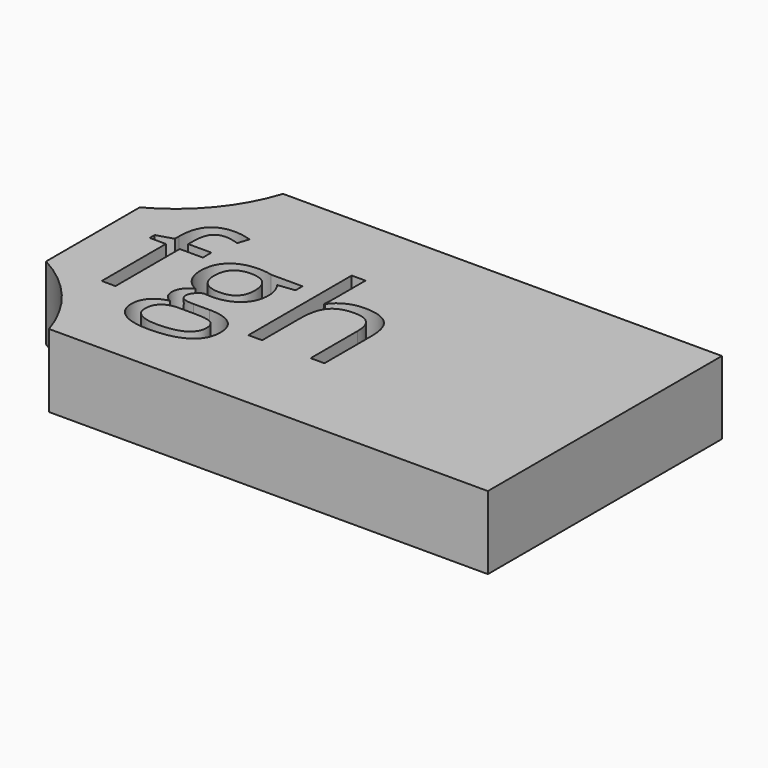
from build123d import *

# Parameters (mm, degrees)
F0_W         = 150
F0_H         = 100
F1_DEPTH     = 2
F2_DEPTH     = 25
F3_TEXT_SIZE = 58.1079033307
F4_DEPTH     = 25


# Not quite as in the source:
# - Text() gives the source's letters only with a copy of the font that has no kerning and outlines rounded to 1/6400 em; it was checked with that copy


with BuildPart() as f1:
    # F0 (on Top) → F1 (new body)
    with BuildSketch(Plane.XY):
        Rectangle(F0_W, F0_H)
    extrude(amount=F1_DEPTH)

    # F0 (on Top) → F2 (join)
    with BuildSketch(Plane.XY):
        Rectangle(F0_W, F0_H)
        with BuildLine():
            Line((-75, -50), (-75, 50))
            ThreePointArc((-75, 50), (-84.5768540724, 32.5640450603), (-100, 20))
            Line((-100, 20), (-100, -20))
            ThreePointArc((-100, -20), (-84.5768540724, -32.5640450603), (-75, -50))
        make_face()
    extrude(amount=F2_DEPTH)

    # F3 (on face) → F4 (cut)
    with BuildSketch(Plane.XY.offset(25)):
        with Locations((-87.7241939306, -19.569247961)):
            Text('fgh', F3_TEXT_SIZE, font='Open Sans', text_align=(TextAlign.LEFT, TextAlign.BOTTOM))
    extrude(amount=-F4_DEPTH, mode=Mode.SUBTRACT)


solid = f1.part
